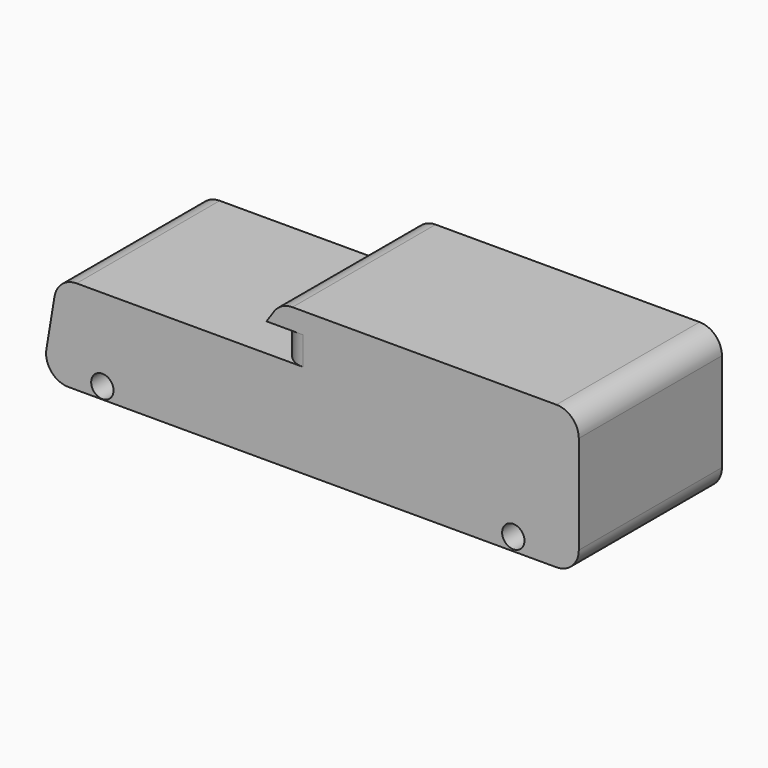
from build123d import *

# Parameters (mm, degrees)
F0_R        = 2.5
F0_W        = 4.0654889308
F0_H        = 4.077391699
F1_DEPTH    = 40
F2_DEPTH    = 0.1
F3_W        = 37.3762528179
F3_H        = 4.5243166387
F4_DEPTH    = 0.8
F5_T1_DEPTH = 61.1957339443
F5_T3_DEPTH = 69.4870657294
F5_T5_DEPTH = 6.3301489651
F5_T7_DEPTH = 53.3325486423
F5_T9_DEPTH = 65


# Not quite as in the source:
# - a fillet or chamfer that OpenCascade refuses, or shapes differently, is made with other operations: its cross-section is extruded or revolved along the edge and cut away or added


with BuildPart() as f1:
    # F0 (on Front) → F1 (new body)
    with BuildSketch(Plane.XZ):
        Polygon((-49.8398691416, 21), (-53.3222284913, 0), (0, 0), (26.6024060547, 0), (66.6777715087, 0), (66.6777715087, 32.0019141734), (0, 32.0019141734), (0, 27.3301489651), (0, 26.5009570867), (4.0654889308, 26.5009570867), (4.0654889308, 22.4235653877), (0, 22.4235653877), (0, 21), align=None)
        with Locations((-39.8388169706, 2.6)):
            Circle(F0_R, mode=Mode.SUBTRACT)
        with Locations((52.0384535193, 2.9)):
            Circle(F0_R, mode=Mode.SUBTRACT)
        with Locations((2.0327444654, 24.4622612372)):
            Rectangle(F0_W, F0_H)
        Polygon((0, 27.3301489651), (0, 32.0019141734), (-3.1343069183, 27.3301489651), align=None)
    extrude(amount=F1_DEPTH)

    # F2 (add): a face of the model
    f2_faces = [f1.faces().sort_by_distance(p)[0] for p in [
        (-24.9199345708, -20, 21),
    ]]
    extrude(f2_faces, amount=-F2_DEPTH)

    # F3 (on Right) → F4 (cut)
    with BuildSketch(Plane.YZ):
        with Locations((-20.0095633627, 24.2089927197)):
            Rectangle(F3_W, F3_H)
    extrude(amount=F4_DEPTH, mode=Mode.SUBTRACT)

    # F5: fillet of radius 5 on 7 edges, made by hand

    # F5_s2 → F5_t1 (cut)
    with BuildSketch(Plane.XZ.offset(-10.5978669722)):
        with BuildLine():
            ThreePointArc((-50.5333622544, 16.81796308), (-48.8341558683, 19.8137786643), (-45.6007223527, 21))
            Line((-45.6007223527, 21), (-49.8398691416, 21))
            Line((-49.8398691416, 21), (-50.5333622544, 16.81796308))
        make_face()
    extrude(amount=F5_T1_DEPTH, mode=Mode.SUBTRACT)

    # F5_s4 → F5_t3 (cut)
    with BuildSketch(Plane.XZ.offset(-14.7435328647)):
        with BuildLine():
            ThreePointArc((-52.3574552471, 5.81796308), (-51.2385940097, 1.7665664844), (-47.4248153454, 0))
            Line((-47.4248153454, 0), (-53.3222284913, 0))
            Line((-53.3222284913, 0), (-52.3574552471, 5.81796308))
        make_face()
    extrude(amount=F5_T3_DEPTH, mode=Mode.SUBTRACT)

    # F5_s6 → F5_t5 (cut)
    with BuildSketch(Plane.XY.offset(21)):
        with BuildLine():
            ThreePointArc((5, 0), (1.4644660941, -1.4644660941), (0, -5))
            Line((0, -5), (0, 0))
            Line((0, 0), (5, 0))
        make_face()
        with BuildLine():
            ThreePointArc((5, -40), (1.4644660941, -38.5355339059), (0, -35))
            Line((0, -35), (0, -40))
            Line((0, -40), (5, -40))
        make_face()
    extrude(amount=F5_T5_DEPTH, mode=Mode.SUBTRACT)

    # F5_s8 → F5_t7 (cut)
    with BuildSketch(Plane.XZ.offset(-6.6662743212)):
        with BuildLine():
            ThreePointArc((2.6665097285, 32.0019141734), (0.3136763633, 31.4137363769), (-1.4856032643, 29.7875842356))
            Line((-1.4856032643, 29.7875842356), (0, 32.0019141734))
            Line((0, 32.0019141734), (2.6665097285, 32.0019141734))
        make_face()
    extrude(amount=F5_T7_DEPTH, mode=Mode.SUBTRACT)

    # F5_s10 → F5_t9 (cut)
    with BuildSketch(Plane.XZ.offset(-12.5)):
        with BuildLine():
            ThreePointArc((61.6777715087, 0), (65.2133054146, 1.4644660941), (66.6777715087, 5))
            Line((66.6777715087, 5), (66.6777715087, 0))
            Line((66.6777715087, 0), (61.6777715087, 0))
        make_face()
        with BuildLine():
            ThreePointArc((66.6777715087, 27.0019141734), (65.2133054146, 30.5374480793), (61.6777715087, 32.0019141734))
            Line((61.6777715087, 32.0019141734), (66.6777715087, 32.0019141734))
            Line((66.6777715087, 32.0019141734), (66.6777715087, 27.0019141734))
        make_face()
    extrude(amount=F5_T9_DEPTH, mode=Mode.SUBTRACT)


solid = f1.part
